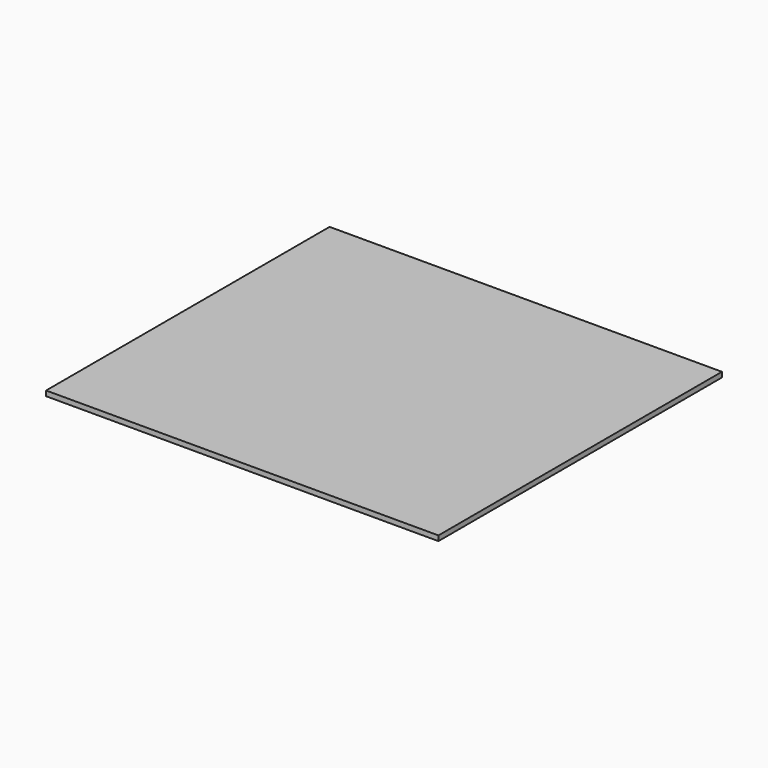
from build123d import *

# Parameters (mm, degrees)
F0_W     = 38.1
F0_H     = 38.1
F0_W_2   = 628.65
F0_H_2   = 812.8
F1_DEPTH = 12.7


with BuildPart() as f1:
    # F0 (on Top) → F1 (new body)
    with BuildSketch(Plane.XY):
        with Locations((142.1793598415, -431.3289260195)):
            Rectangle(F0_W, F0_H)
        Polygon((161.2293598415, 399.428513117), (161.2293598415, -412.2789260195), (161.2293598415, -450.3789260195), (440.6293598415, -450.3789260195), (440.6293598415, 438.6210739805), (161.2293598415, 438.6210739805), (161.2293598415, 400.5210739805), align=None)
        Polygon((123.1293598415, -412.2789260195), (161.2293598415, -412.2789260195), (161.2293598415, 399.428513117), (161.2293598415, 400.5210739805), (123.1293598415, 400.5210739805), align=None)
        Polygon((123.1293598415, -450.3789260195), (123.1293598415, -412.2789260195), (-505.5206401585, -412.2789260195), (-505.5206401585, -450.3789260195), (-488.6698754547, -450.3789260195), align=None)
        with Locations((-191.1956401585, -5.8789260195)):
            Rectangle(F0_W_2, F0_H_2)
        with Locations((-524.5706401585, -431.3289260195)):
            Rectangle(F0_W, F0_H)
        with Locations((-524.5706401585, -5.8789260195)):
            Rectangle(F0_W, F0_H_2)
        with Locations((-191.1956401585, 419.5710739805)):
            Rectangle(F0_W_2, F0_H)
        with Locations((142.1793598415, 419.5710739805)):
            Rectangle(F0_W, F0_H)
        with Locations((-524.5706401585, 419.5710739805)):
            Rectangle(F0_W, F0_H)
    extrude(amount=F1_DEPTH)


solid = f1.part
